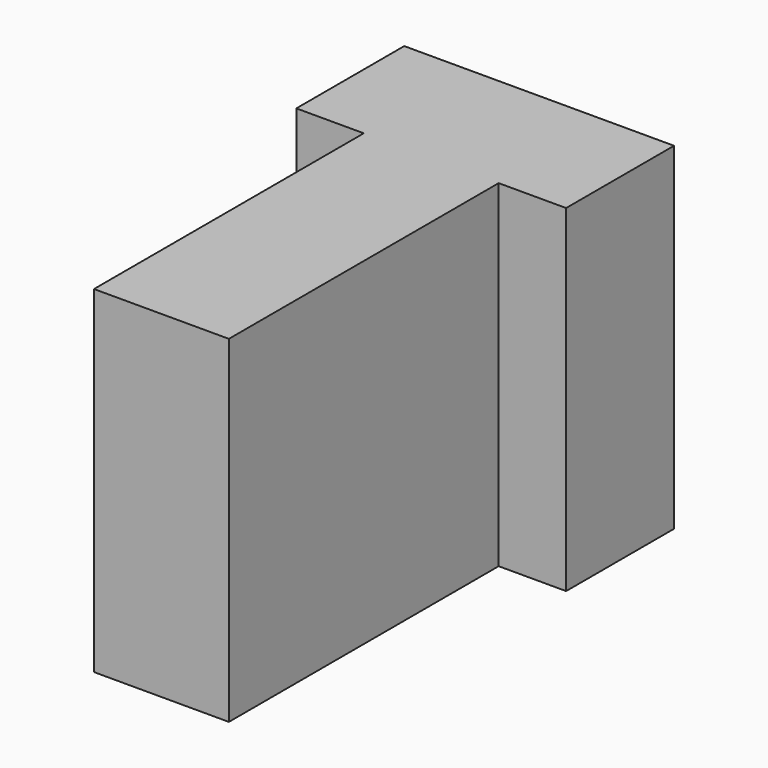
from build123d import *

# Parameters (mm, degrees)
F1_DEPTH = 31.75


# Not quite as in the source:
# - a length typed as a fraction of an inch, garbled in the dataset ("3 / 203.2 mm" for 3/8 in), is restored


with BuildPart() as f1:
    # F0 (on Top) → F1 (new body)
    with BuildSketch(Plane.XY):
        Polygon((11.9089967117, 44.45), (0, 44.45), (-13.4910032883, 44.45), (-13.4910032883, 31.75), (-7.1410032883, 31.75), (-7.1410032883, 0), (5.5589967117, 0), (5.5589967117, 31.75), (11.9089967117, 31.75), align=None)
    extrude(amount=F1_DEPTH)


solid = f1.part
